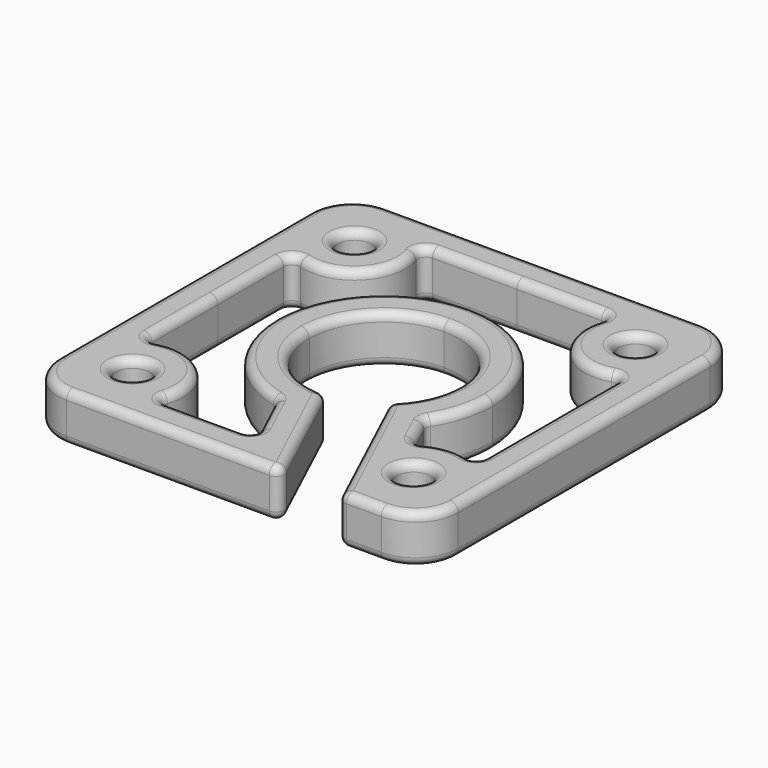
from build123d import *

# Parameters (mm, degrees)
F0_R     = 3.175
F1_DEPTH = 9
F2_R     = 1.5625
F3_R     = 1.5625


# Not quite as in the source:
# - ends of sketch curves that miss each other by under 0.0002 mm in the source are joined


with BuildPart() as f1:
    # F0 (on Top) → F1 (new body)
    with BuildSketch(Plane.XY):
        with BuildLine():
            Line((0, 31.15), (0, 37.5))
            Line((0, 37.5), (-29.5, 37.5))
            ThreePointArc((-29.5, 37.5), (-35.1568542495, 35.1568542495), (-37.5, 29.5))
            Line((-37.5, 29.5), (-37.5, 0))
            Line((-37.5, 0), (-31.15, 0))
            Line((-31.15, 0), (-31.15, 17.787572))
            ThreePointArc((-31.15, 17.787572), (-19.4562116609, 19.400996919), (-18.3122078194, 31.1500001161))
            Line((-18.3122078194, 31.1500001161), (0, 31.15))
        make_face()
        with Locations((-26.324893, 26)):
            Circle(F0_R, mode=Mode.SUBTRACT)
        with BuildLine():
            Line((29.5, 37.5), (0, 37.5))
            Line((0, 37.5), (0, 31.15))
            Line((0, 31.15), (18.312208, 31.15))
            ThreePointArc((18.312208, 31.15), (19.4562116609, 19.400996919), (31.1499998347, 17.7875722814))
            Line((31.1499998347, 17.7875722814), (31.15, 0))
            Line((31.15, 0), (37.5, 0))
            Line((37.5, 0), (37.5, 29.5))
            ThreePointArc((37.5, 29.5), (35.1568542495, 35.1568542495), (29.5, 37.5))
        make_face()
        with Locations((26.324893, 26)):
            Circle(F0_R, mode=Mode.SUBTRACT)
        with BuildLine():
            ThreePointArc((16.8397715275, -11.4256113579), (19.4526585662, -5.9763345545), (20.35, 0))
            Line((20.35, 0), (14, 0))
            ThreePointArc((14, 0), (12.787539009, -5.6990215031), (9.3601648439, -10.4109228263))
            Line((9.3601648439, -10.4109228263), (21.992009, -37.5))
            Line((21.992009, -37.5), (29.5, -37.5))
            ThreePointArc((29.5, -37.5), (35.1568542495, -35.1568542495), (37.5, -29.5))
            Line((37.5, -29.5), (37.5, 0))
            Line((37.5, 0), (31.15, 0))
            Line((31.15, 0), (31.15, -17.787572))
            ThreePointArc((31.15, -17.787572), (25.5453777615, -16.5069509117), (20.2247368228, -18.6846927875))
            Line((20.2247368228, -18.6846927875), (16.8397715275, -11.4256113579))
        make_face()
        with Locations((26.324893, -26)):
            Circle(F0_R, mode=Mode.SUBTRACT)
        with BuildLine():
            Line((-14, 0), (-20.35, 0))
            ThreePointArc((-20.35, 0), (-15.822690769, -12.7970682903), (-4.2551639482, -19.9001527576))
            Line((-4.2551639482, -19.9001527576), (0, -29.025381314))
            Line((0, -29.025381314), (0, -14))
            ThreePointArc((0, -14), (-9.8994949366, -9.8994949366), (-14, 0))
        make_face()
        with BuildLine():
            ThreePointArc((20.35, 0), (14.3896229971, 14.3896229971), (0, 20.35))
            Line((0, 20.35), (0, 14))
            ThreePointArc((0, 14), (9.8994949366, 9.8994949366), (14, 0))
            Line((14, 0), (20.35, 0))
        make_face()
        with BuildLine():
            Line((0, 14), (0, 20.35))
            ThreePointArc((0, 20.35), (-14.3896229971, 14.3896229971), (-20.35, 0))
            Line((-20.35, 0), (-14, 0))
            ThreePointArc((-14, 0), (-9.8994949366, 9.8994949366), (0, 14))
        make_face()
        with BuildLine():
            Line((-31.15, 0), (-37.5, 0))
            Line((-37.5, 0), (-37.5, -29.5))
            ThreePointArc((-37.5, -29.5), (-35.1568542495, -35.1568542495), (-29.5, -37.5))
            Line((-29.5, -37.5), (0, -37.5))
            Line((0, -37.5), (0, -31.15))
            Line((0, -31.15), (-18.312208, -31.15))
            ThreePointArc((-18.312208, -31.15), (-19.4562116609, -19.400996919), (-31.1499998347, -17.7875722814))
            Line((-31.1499998347, -17.7875722814), (-31.15, 0))
        make_face()
        with Locations((-26.324893, -26)):
            Circle(F0_R, mode=Mode.SUBTRACT)
        Polygon((10.95823, -37.5), (0, -14), (0, -29.025381314), (0.990726, -31.15), (0, -31.15), (0, -37.5), align=None)
    extrude(amount=F1_DEPTH)

    # F2
    f2_edges = [f1.edges().sort_by_distance(p)[0] for p in [
        (9.360165, -10.410923, 4.5),
        (0, -14, 4.5),
        (16.839772, -11.425611, 4.5),
        (-4.255164, -19.900153, 4.5),
        (21.992009, -37.5, 4.5),
        (10.95823, -37.5, 4.5),
        (31.15, 17.787572, 4.5),
        (18.312208, 31.15, 4.5),
        (-18.312208, 31.15, 4.5),
        (20.224737, -18.684693, 4.5),
        (-31.15, -17.787572, 4.5),
        (-18.312208, -31.15, 4.5),
        (31.15, -17.787572, 4.5),
        (-31.15, 17.787572, 4.5),
        (0.990726, -31.15, 4.5),
    ]]
    fillet(f2_edges, radius=F2_R)

    # F3
    f3_edges = [f1.edges().sort_by_distance(p)[0] for p in [
        (-7.916913, 31.15, 0),
        (-17.104918, 30.496197, 0),
        (7.916913, 31.15, 0),
        (-19.486745, 19.369362, 0),
        (17.104918, 30.496196, 0),
        (-30.51567, 16.660338, 0),
        (19.486745, 19.369362, 0),
        (-31.15, 7.701697, 0),
        (30.51567, 16.660338, 0),
        (-31.15, -7.701697, 0),
        (31.15, 7.701697, 0),
        (-30.51567, -16.660338, 0),
        (31.15, -7.701697, 0),
        (-19.486745, -19.369362, 0),
        (30.51567, -16.660338, 0),
        (-17.104918, -30.496196, 0),
        (25.295307, -16.530809, 0),
        (-8.647867, -31.15, 0),
        (20.385073, -17.840433, 0),
        (-0.144109, -30.427031, 0),
        (18.325257, -14.611246, 0),
        (-1.989875, -24.75808, 0),
        (17.061871, -11.456817, 0),
        (-4.354795, -20.044825, 0),
        (-7.633097, 18.864208, 0),
        (-29.499893, 26, 0),
        (23.149893, 26, 0),
        (23.149893, -26, 0),
        (-29.499893, -26, 0),
        (-5.079542, 13.046005, 0),
        (-0.12884, -14.239816, 0),
        (9.704119, -10.503247, 0),
        (5.163532, -25.07323, 0),
        (15.700508, -24.007833, 0),
        (9.823395, -36.777031, 0),
        (22.147901, -37.255299, 0),
        (-10.497202, -37.5, 0),
        (26.243716, -37.5, 0),
        (-35.156854, -35.156854, 0),
        (35.156854, -35.156854, 0),
        (-37.5, 0, 0),
        (37.5, 0, 0),
        (-35.156854, 35.156854, 0),
        (35.156854, 35.156854, 0),
        (0, 37.5, 0),
        (-7.916913, 31.15, 9),
        (-17.104918, 30.496197, 9),
        (7.916913, 31.15, 9),
        (-19.486745, 19.369362, 9),
        (17.104918, 30.496196, 9),
        (-30.51567, 16.660338, 9),
        (19.486745, 19.369362, 9),
        (-31.15, 7.701697, 9),
        (30.51567, 16.660338, 9),
        (-31.15, -7.701697, 9),
        (31.15, 7.701697, 9),
        (-30.51567, -16.660338, 9),
        (31.15, -7.701697, 9),
        (-19.486745, -19.369362, 9),
        (30.51567, -16.660338, 9),
        (-17.104918, -30.496196, 9),
        (25.295307, -16.530809, 9),
        (-8.647867, -31.15, 9),
        (20.385073, -17.840433, 9),
        (-0.144109, -30.427031, 9),
        (18.325257, -14.611246, 9),
        (-1.989875, -24.75808, 9),
        (17.061871, -11.456817, 9),
        (-4.354795, -20.044825, 9),
        (-7.633097, 18.864208, 9),
        (-29.499893, 26, 9),
        (23.149893, 26, 9),
        (23.149893, -26, 9),
        (-29.499893, -26, 9),
        (-5.079542, 13.046005, 9),
        (-0.12884, -14.239816, 9),
        (9.704119, -10.503247, 9),
        (5.163532, -25.07323, 9),
        (15.700508, -24.007833, 9),
        (9.823395, -36.777031, 9),
        (22.147901, -37.255299, 9),
        (-10.497202, -37.5, 9),
        (26.243716, -37.5, 9),
        (-35.156854, -35.156854, 9),
        (35.156854, -35.156854, 9),
        (-37.5, 0, 9),
        (37.5, 0, 9),
        (-35.156854, 35.156854, 9),
        (35.156854, 35.156854, 9),
        (0, 37.5, 9),
    ]]
    fillet(f3_edges, radius=F3_R)


solid = f1.part
